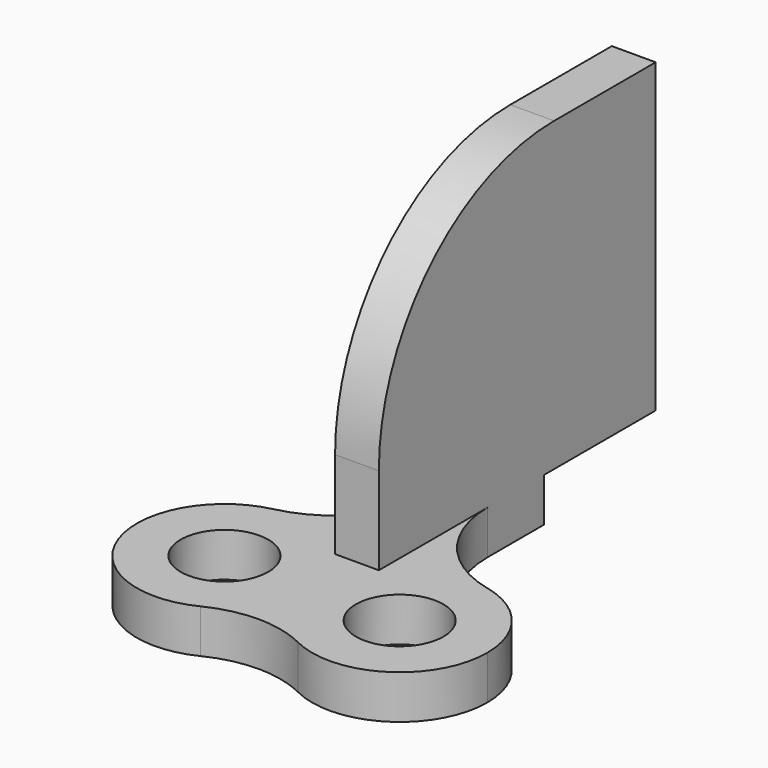
from build123d import *

# Parameters (mm, degrees)
F0_R     = 10
F1_DEPTH = 10
F2_R     = 25
F3_R     = 25
F4_W     = 10
F4_H     = 79.0000073612
F5_DEPTH = 70
F6_R     = 50


with BuildPart() as f1:
    # F0 (on Top) → F1 (new body)
    with BuildSketch(Plane.XY):
        with BuildLine():
            Line((-5, 10.7507640496), (0, 10.7507640496))
            ThreePointArc((0, 10.7507640496), (-1.2917130661, 17.8218318615), (-5, 23.9795206049))
            Line((-5, 23.9795206049), (-5, 10.7507640496))
        make_face()
        with BuildLine():
            Line((5, 10.7507640496), (0, 10.7507640496))
            ThreePointArc((0, 10.7507640496), (20, -9.2492359504), (40, 10.7507640496))
            ThreePointArc((40, 10.7507640496), (27.0710678119, 29.4590509835), (5, 23.9795206049))
            Line((5, 23.9795206049), (5, 10.7507640496))
        make_face()
        with Locations((20, 10.7507640496)):
            Circle(F0_R, mode=Mode.SUBTRACT)
        with BuildLine():
            ThreePointArc((-5, 23.9795206049), (-1.2917130661, 17.8218318615), (0, 10.7507640496))
            ThreePointArc((0, 10.7507640496), (1.2917130661, 17.8218318615), (5, 23.9795206049))
            Line((5, 23.9795206049), (5, 70.7507640496))
            Line((5, 70.7507640496), (-5, 70.7507640496))
            Line((-5, 70.7507640496), (-5, 23.9795206049))
        make_face()
        with BuildLine():
            ThreePointArc((-5, 23.9795206049), (-38.7082869339, 3.6796962377), (0, 10.7507640496))
            Line((0, 10.7507640496), (-5, 10.7507640496))
            Line((-5, 10.7507640496), (-5, 23.9795206049))
        make_face()
        with Locations((-20, 10.7507640496)):
            Circle(F0_R, mode=Mode.SUBTRACT)
        with BuildLine():
            ThreePointArc((5, 23.9795206049), (1.2917130661, 17.8218318615), (0, 10.7507640496))
            Line((0, 10.7507640496), (5, 10.7507640496))
            Line((5, 10.7507640496), (5, 23.9795206049))
        make_face()
    extrude(amount=F1_DEPTH)

    # F2
    f2_edges = [f1.edges().sort_by_distance(p)[0] for p in [
        (0, 10.750764, 5),
    ]]
    fillet(f2_edges, radius=F2_R)

    # F3
    f3_edges = [f1.edges().sort_by_distance(p)[0] for p in [
        (-5, 23.979521, 5),
        (5, 23.979521, 5),
    ]]
    fillet(f3_edges, radius=F3_R)

    # F4 (on face) → F5 (join)
    with BuildSketch(Plane.XY.offset(10)):
        with Locations((0, 63.0660597235)):
            Rectangle(F4_W, F4_H)
    extrude(amount=F5_DEPTH)

    # F6
    f6_edges = [f1.edges().sort_by_distance(p)[0] for p in [
        (0, 23.566056, 80),
    ]]
    fillet(f6_edges, radius=F6_R)


solid = f1.part
